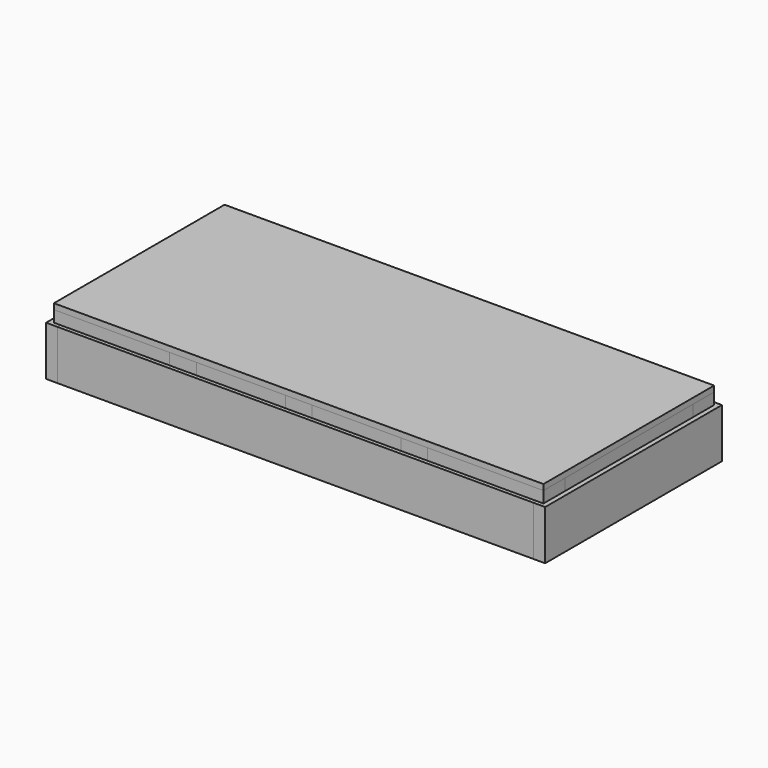
from build123d import *

# Parameters (mm, degrees)
F1_DEPTH  = 82.55
F0_W      = 1587.5
F0_H      = 38.1
F2_DEPTH  = 82.55
F3_DEPTH  = 82.55
F4_DEPTH  = 82.55
F5_W      = 88.9
F5_H      = 533.4
F6_DEPTH  = 38.1
F5_H_2    = 25.4
F7_DEPTH  = 38.1
F8_DEPTH  = 38.1
F9_DEPTH  = 38.1
F10_DEPTH = 38.1
F11_DEPTH = 38.1
F5_W_2    = 296.8625
F5_H_3    = 88.9
F5_W_3    = 363.5375
F12_DEPTH = 38.1
F5_H_4    = 63.5
F15_W     = 1631.95
F15_H     = 711.2
F16_DEPTH = 19.05


# Not quite as in the source:
# - a feature names something its author has since deleted; it is built from what else it names


with BuildPart() as f1:
    # F0 (on Top) → F1 (new body, symmetric)
    with BuildSketch(Plane.XY):
        Polygon((0, -38.1), (0, 0), (0, 660.4), (0, 698.5), (-38.1, 698.5), (-38.1, -38.1), align=None)
    extrude(amount=F1_DEPTH, both=True)


with BuildPart() as f2:
    # F0 (on Top) → F2 (new body, symmetric)
    with BuildSketch(Plane.XY):
        with Locations((793.75, 679.45)):
            Rectangle(F0_W, F0_H)
    extrude(amount=F2_DEPTH, both=True)


with BuildPart() as f3:
    # F0 (on Top) → F3 (new body, symmetric)
    with BuildSketch(Plane.XY):
        with Locations((793.75, -19.05)):
            Rectangle(F0_W, F0_H)
    extrude(amount=F3_DEPTH, both=True)


with BuildPart() as f4:
    # F0 (on Top) → F4 (new body, symmetric)
    with BuildSketch(Plane.XY):
        Polygon((1587.5, 660.4), (1587.5, 0), (1587.5, -38.1), (1625.6, -38.1), (1625.6, 698.5), (1587.5, 698.5), align=None)
    extrude(amount=F4_DEPTH, both=True)


with BuildPart() as f6:
    # F5 (on face) → F6 (new body)
    with BuildSketch(Plane.XY.offset(82.55)):
        with Locations((22.225, 330.2)):
            Rectangle(F5_W, F5_H)
    extrude(amount=F6_DEPTH)


with BuildPart() as f7:
    # F5 (on face) → F7 (new body)
    with BuildSketch(Plane.XY.offset(82.55)):
        Polygon((363.5375, 596.9), (363.5375, 63.5), (363.5375, 0), (452.4375, 0), (452.4375, 63.5), (452.4375, 596.9), (452.4375, 685.8), (363.5375, 685.8), align=None)
        with Locations((407.9875, -12.7)):
            Rectangle(F5_W, F5_H_2)
    extrude(amount=F7_DEPTH)


with BuildPart() as f8:
    # F5 (on face) → F8 (new body)
    with BuildSketch(Plane.XY.offset(82.55)):
        Polygon((749.3, 63.5), (749.3, 0), (838.2, 0), (838.2, 63.5), (838.2, 596.9), (838.2, 685.8), (749.3, 685.8), (749.3, 596.9), align=None)
        with Locations((793.75, -12.7)):
            Rectangle(F5_W, F5_H_2)
    extrude(amount=F8_DEPTH)


with BuildPart() as f9:
    # F5 (on face) → F9 (new body)
    with BuildSketch(Plane.XY.offset(82.55)):
        Polygon((1135.0625, 0), (1223.9625, 0), (1223.9625, 63.5), (1223.9625, 596.9), (1223.9625, 685.8), (1135.0625, 685.8), (1135.0625, 596.9), (1135.0625, 63.5), align=None)
        with Locations((1179.5125, -12.7)):
            Rectangle(F5_W, F5_H_2)
    extrude(amount=F9_DEPTH)


with BuildPart() as f10:
    # F5 (on face) → F10 (new body)
    with BuildSketch(Plane.XY.offset(82.55)):
        with Locations((1565.275, 330.2)):
            Rectangle(F5_W, F5_H)
    extrude(amount=F10_DEPTH)


with BuildPart() as f11:
    # F5 (on face) → F11 (new body)
    with BuildSketch(Plane.XY.offset(82.55)):
        Polygon((-22.225, 685.8), (-22.225, 596.9), (66.675, 596.9), (363.5375, 596.9), (363.5375, 685.8), align=None)
    extrude(amount=F11_DEPTH)


with BuildPart() as f11b:
    # F5 (on face) → F11, piece 2 (new body)
    with BuildSketch(Plane.XY.offset(82.55)):
        with Locations((600.86875, 641.35)):
            Rectangle(F5_W_2, F5_H_3)
    extrude(amount=F11_DEPTH)


with BuildPart() as f11c:
    # F5 (on face) → F11, piece 3 (new body)
    with BuildSketch(Plane.XY.offset(82.55)):
        with Locations((986.63125, 641.35)):
            Rectangle(F5_W_2, F5_H_3)
    extrude(amount=F11_DEPTH)


with BuildPart() as f11d:
    # F5 (on face) → F11, piece 4 (new body)
    with BuildSketch(Plane.XY.offset(82.55)):
        Polygon((1520.825, 596.9), (1609.725, 596.9), (1609.725, 685.8), (1223.9625, 685.8), (1223.9625, 596.9), align=None)
    extrude(amount=F11_DEPTH)


with BuildPart() as f12:
    # F5 (on face) → F12 (new body)
    with BuildSketch(Plane.XY.offset(82.55)):
        with Locations((181.76875, -12.7)):
            Rectangle(F5_W_3, F5_H_2)
        Polygon((-22.225, 63.5), (-22.225, -25.4), (0, -25.4), (0, 0), (363.5375, 0), (363.5375, 63.5), (66.675, 63.5), align=None)
    extrude(amount=F12_DEPTH)


with BuildPart() as f12b:
    # F5 (on face) → F12, piece 2 (new body)
    with BuildSketch(Plane.XY.offset(82.55)):
        with Locations((600.86875, 31.75)):
            Rectangle(F5_W_2, F5_H_4)
        with Locations((600.86875, -12.7)):
            Rectangle(F5_W_2, F5_H_2)
    extrude(amount=F12_DEPTH)


with BuildPart() as f12c:
    # F5 (on face) → F12, piece 3 (new body)
    with BuildSketch(Plane.XY.offset(82.55)):
        with Locations((986.63125, 31.75)):
            Rectangle(F5_W_2, F5_H_4)
        with Locations((986.63125, -12.7)):
            Rectangle(F5_W_2, F5_H_2)
    extrude(amount=F12_DEPTH)


with BuildPart() as f12d:
    # F5 (on face) → F12, piece 4 (new body)
    with BuildSketch(Plane.XY.offset(82.55)):
        Polygon((1587.5, 0), (1587.5, -25.4), (1609.725, -25.4), (1609.725, 63.5), (1520.825, 63.5), (1223.9625, 63.5), (1223.9625, 0), align=None)
        with Locations((1405.73125, -12.7)):
            Rectangle(F5_W_3, F5_H_2)
    extrude(amount=F12_DEPTH)


with BuildPart() as f16:
    # F15 (on 3pt) → F16 (new body)
    with BuildSketch(Plane(origin=(0, 0, 120.65), x_dir=(1, 0, 0), z_dir=(0, 0, -1))):
        with Locations((793.75, -330.2)):
            Rectangle(F15_W, F15_H)
    extrude(amount=-F16_DEPTH)


solid = Compound([f1.part, f2.part, f3.part, f4.part, f6.part, f7.part, f8.part, f9.part, f10.part, f11.part, f11b.part, f11c.part, f11d.part, f12.part, f12b.part, f12c.part, f12d.part, f16.part])
